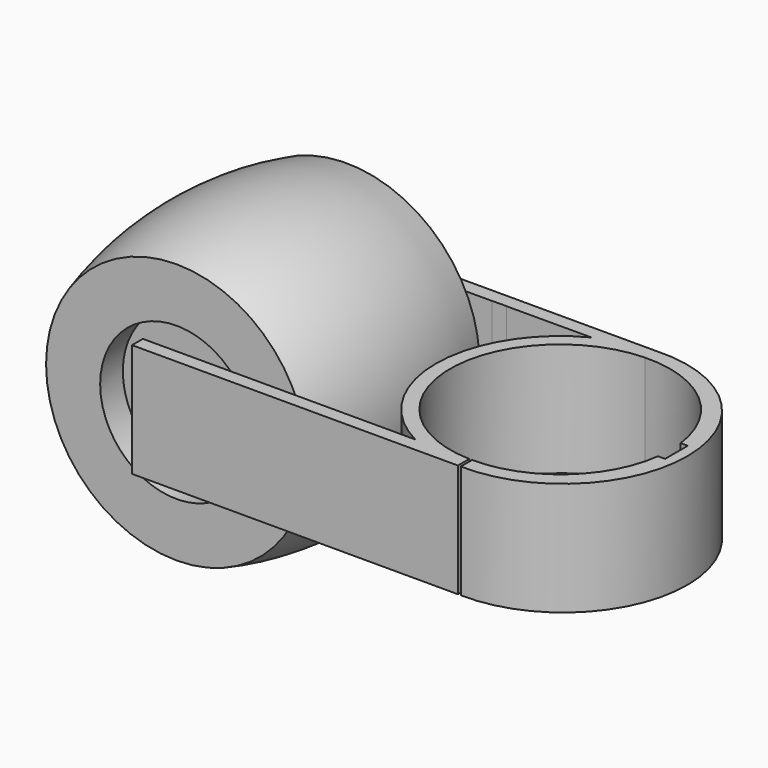
from build123d import *

# Parameters (mm, degrees)
F1_DEPTH = 25.4
F2_DEPTH = 0.254
F0_W     = 27.8709288151
F0_H     = 69.85
F3_DEPTH = 0.254
F5_DEPTH = 3.175
F6_DEPTH = 25.4


# Not quite as in the source:
# - the program builds the solid bodies; features that only make, move or delete a surface that nothing else refers to are left out


with BuildPart() as f1:
    # F0 (on Top) → F1 (new body, symmetric)
    with BuildSketch(Plane.XY):
        with BuildLine():
            ThreePointArc((-1.2680592233, -49.1961602369), (-49.2125, 0), (-1.2680592233, 49.1961602369))
            Line((-1.2680592233, 49.1961602369), (-1.2680592233, 55.5480281563))
            Line((-1.2680592233, 55.5480281563), (-147.3180592233, 55.5480281563))
            Line((-147.3180592233, 55.5480281563), (-147.3180592233, 49.091055685))
            Line((-147.3180592233, 49.091055685), (-69.8634971885, 49.2936872058))
            Line((-69.8634971885, 49.2936872058), (-63.5134971885, 49.4099743665))
            ThreePointArc((-63.5134971885, 49.4099743665), (-63.4974587718, 49.3601815353), (-63.4814364191, 49.3103835326))
            Line((-63.4814364191, 49.3103835326), (-25.4134971885, 49.4099743665))
            ThreePointArc((-25.4134971885, 49.4099743665), (-55.5624058885, -0.1022650226), (-25.2314432137, -49.5031885802))
            Line((-25.2314432137, -49.5031885802), (-63.3314432137, -49.5031885802))
            Line((-63.3314432137, -49.5031885802), (-69.6814432137, -49.5031885802))
            Line((-69.6814432137, -49.5031885802), (-147.3180592233, -49.5031885802))
            Line((-147.3180592233, -49.5031885802), (-147.3180592233, -55.5800534785))
            Line((-147.3180592233, -55.5800534785), (-1.2680592233, -55.5800534785))
            Line((-1.2680592233, -55.5800534785), (-1.2680592233, -49.1961602369))
        make_face()
    extrude(amount=F1_DEPTH, both=True)

    # F0 (on Top) → F5 (join, symmetric)
    with BuildSketch(Plane.XY):
        with BuildLine():
            ThreePointArc((49.0389416617, -6.35), (32.6236991353, -37.0532891725), (0, -49.2125))
            Line((0, -49.2125), (0, -55.5625))
            ThreePointArc((0, -55.5625), (57.0543020001, 0.6511375212), (-1.2680592233, 55.5480281563))
            Line((-1.2680592233, 55.5480281563), (-1.2680592233, 49.1961602369))
            ThreePointArc((-1.2680592233, 49.1961602369), (32.1458766832, 37.4716025001), (49.0397283671, 6.35))
            Line((49.0397283671, 6.35), (52.2147283671, 6.35))
            Line((52.2147283671, 6.35), (52.2147283671, -6.35))
            Line((52.2147283671, -6.35), (49.0389416617, -6.35))
        make_face()
        with BuildLine():
            Line((-25.4134971885, 49.4099743665), (-63.4814364191, 49.3103835326))
            ThreePointArc((-63.4814364191, 49.3103835326), (-55.6963964132, -0.0846991302), (-63.3314432137, -49.5031885802))
            Line((-63.3314432137, -49.5031885802), (-25.2314432137, -49.5031885802))
            ThreePointArc((-25.2314432137, -49.5031885802), (-55.5624058885, -0.1022650226), (-25.4134971885, 49.4099743665))
        make_face()
    extrude(amount=F5_DEPTH, both=True)

    # F0 (on Top) → F6 (join, symmetric)
    with BuildSketch(Plane.XY):
        with BuildLine():
            ThreePointArc((49.0389416617, -6.35), (32.6236991353, -37.0532891725), (0, -49.2125))
            Line((0, -49.2125), (0, -55.5625))
            ThreePointArc((0, -55.5625), (57.0543020001, 0.6511375212), (-1.2680592233, 55.5480281563))
            Line((-1.2680592233, 55.5480281563), (-1.2680592233, 49.1961602369))
            ThreePointArc((-1.2680592233, 49.1961602369), (32.1458766832, 37.4716025001), (49.0397283671, 6.35))
            Line((49.0397283671, 6.35), (52.2147283671, 6.35))
            Line((52.2147283671, 6.35), (52.2147283671, -6.35))
            Line((52.2147283671, -6.35), (49.0389416617, -6.35))
        make_face()
    extrude(amount=F6_DEPTH, both=True)


with BuildPart() as f2:
    # F0 (on Top) → F2 (new body)
    with BuildSketch(Plane.XY):
        with BuildLine():
            Line((-167.7432940599, 47.3424206634), (-193.1432940599, 47.3424206634))
            ThreePointArc((-193.1432940599, 47.3424206634), (-199.0600226604, -0.3618224561), (-191.9816406704, -47.9075793366))
            Line((-191.9816406704, -47.9075793366), (-167.7432940599, -47.9075793366))
            Line((-167.7432940599, -47.9075793366), (-167.7432940599, -35.2075793366))
            Line((-167.7432940599, -35.2075793366), (-161.3932940599, -35.2075793366))
            Line((-161.3932940599, -35.2075793366), (-161.3932940599, 34.6424206634))
            Line((-161.3932940599, 34.6424206634), (-167.7432940599, 34.6424206634))
            Line((-167.7432940599, 34.6424206634), (-167.7432940599, 47.3424206634))
        make_face()
    extrude(amount=F2_DEPTH)

    # F0 (on Top) → F3 (join)
    with BuildSketch(Plane.XY):
        with Locations((-147.4578296524, -0.2825793366)):
            Rectangle(F0_W, F0_H)
    extrude(amount=F3_DEPTH)


with BuildPart() as f4:
    # F2_face (on face) → F4 (revolve)
    with BuildSketch(Plane(origin=(-167.7046477671, -0.1151986196, 0.254), x_dir=(1, 0, 0), z_dir=(0, 0, 1))):
        with BuildLine():
            Line((34.1822825223, 34.7576192829), (-0.0386462928, 34.7576192829))
            Line((-0.0386462928, 34.7576192829), (-0.0386462928, 47.4576192829))
            Line((-0.0386462928, 47.4576192829), (-25.4386462928, 47.4576192829))
            ThreePointArc((-25.4386462928, 47.4576192829), (-31.3553748933, -0.2466238366), (-24.2769929033, -47.7923807171))
            Line((-24.2769929033, -47.7923807171), (-0.0386462928, -47.7923807171))
            Line((-0.0386462928, -47.7923807171), (-0.0386462928, -35.0923807171))
            Line((-0.0386462928, -35.0923807171), (34.1822825223, -35.0923807171))
            Line((34.1822825223, -35.0923807171), (34.1822825223, 34.7576192829))
        make_face()
    revolve(axis=Axis((-133.5223652449, -0.2825793366, 0.254), (0, -1, 0)))


solid = Compound([f1.part, f2.part, f4.part])
